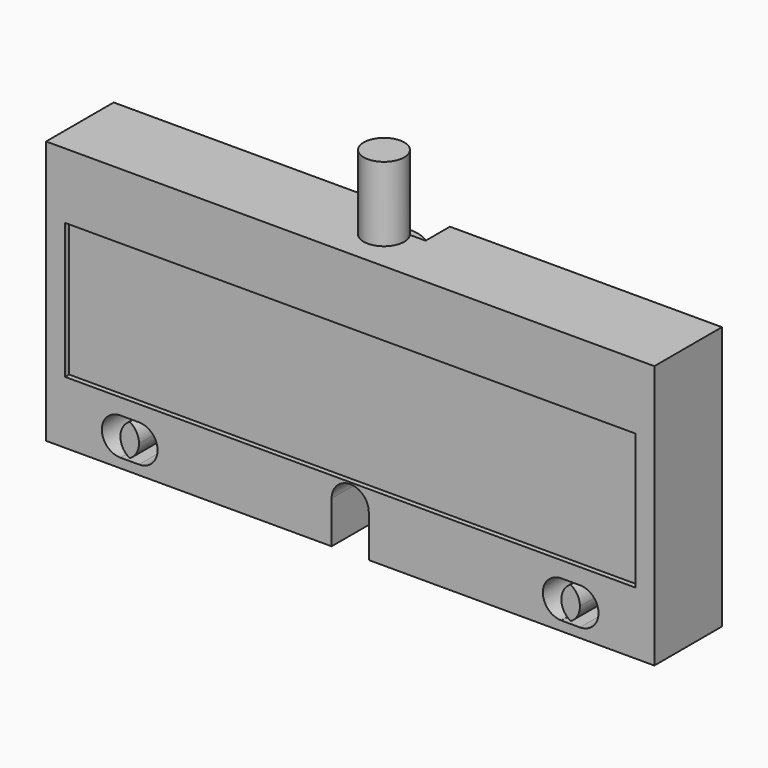
from build123d import *

# Parameters (mm, degrees)
F0_R      = 1.524
F2_DEPTH  = 6.35
F1_R      = 2.54
F3_DEPTH  = 10.16
F4_W      = 45.72
F4_H      = 6.35
F5_DEPTH  = 13.97
F6_DEPTH  = 0.762
F7_DEPTH  = 10.16
F8_DEPTH  = 1.27
F9_DEPTH  = 5.08
F11_DEPTH = 25.4
F12_W     = 21.4504245669
F12_H     = 10.1925823838
F12_W_2   = 21.4354675263
F13_DEPTH = 0.381
F14_W     = 4.826
F14_H     = 20.32
F15_DEPTH = 2.286


with BuildPart() as f2:
    # F0 (on Top) → F2 (new body)
    with BuildSketch(Plane.XY):
        Circle(F0_R)
    extrude(amount=F2_DEPTH)

    # F1 (on Top) → F3 (join)
    with BuildSketch(Plane.XY):
        Circle(F1_R)
    extrude(amount=-F3_DEPTH)


with BuildPart() as f5:
    # F4 (on Top) → F5 (new body)
    with BuildSketch(Plane.XY):
        Rectangle(F4_W, F4_H)
    extrude(amount=-F5_DEPTH)

    # F6 (add): a face of the model
    f6_faces = [f5.faces().sort_by_distance(p)[0] for p in [
        (0, 0, 0),
    ]]
    extrude(f6_faces, amount=F6_DEPTH)

    # F1 (on Top) → F7 (cut)
    with BuildSketch(Plane.XY):
        Circle(F1_R)
    extrude(amount=-F7_DEPTH, mode=Mode.SUBTRACT)

    # F0 (on Top) → F8 (cut)
    with BuildSketch(Plane.XY):
        Circle(F0_R)
    extrude(amount=F8_DEPTH, mode=Mode.SUBTRACT)

    # F9 (add): a face of the model
    f9_faces = [f5.faces().sort_by_distance(p)[0] for p in [
        (0, 0, -13.97),
    ]]
    extrude(f9_faces, amount=F9_DEPTH)

    # F10 (on face) → F11 (cut)
    with BuildSketch(Plane.XZ.offset(3.175)):
        with BuildLine():
            ThreePointArc((-15.875, -18.3439323009), (-14.8871718267, -17.9347604742), (-14.478, -16.9469323009))
            ThreePointArc((-14.478, -16.9469323009), (-14.8871718267, -15.9591041276), (-15.875, -15.5499323009))
            ThreePointArc((-15.875, -15.5499323009), (-16.236570206, -15.5975339216), (-16.5735, -15.7370948118))
            ThreePointArc((-16.5735, -15.7370948118), (-16.0621625109, -16.2484323009), (-15.875, -16.9469323009))
            ThreePointArc((-15.875, -16.9469323009), (-16.0621625109, -17.6454323009), (-16.5735, -18.15676979))
            ThreePointArc((-16.5735, -18.15676979), (-16.236570206, -18.2963306803), (-15.875, -18.3439323009))
        make_face()
        with BuildLine():
            ThreePointArc((-16.5735, -15.7370948118), (-16.236570206, -15.5975339216), (-15.875, -15.5499323009))
            Line((-15.875, -15.5499323009), (-17.272, -15.5499323009))
            ThreePointArc((-17.272, -15.5499323009), (-16.910429794, -15.5975339216), (-16.5735, -15.7370948118))
        make_face()
        with BuildLine():
            Line((-17.272, -18.3439323009), (-15.875, -18.3439323009))
            ThreePointArc((-15.875, -18.3439323009), (-16.236570206, -18.2963306803), (-16.5735, -18.15676979))
            ThreePointArc((-16.5735, -18.15676979), (-16.910429794, -18.2963306803), (-17.272, -18.3439323009))
        make_face()
        with BuildLine():
            ThreePointArc((-16.5735, -18.15676979), (-17.272, -16.9469323009), (-16.5735, -15.7370948118))
            ThreePointArc((-16.5735, -15.7370948118), (-16.910429794, -15.5975339216), (-17.272, -15.5499323009))
            ThreePointArc((-17.272, -15.5499323009), (-18.669, -16.9469323009), (-17.272, -18.3439323009))
            ThreePointArc((-17.272, -18.3439323009), (-16.910429794, -18.2963306803), (-16.5735, -18.15676979))
        make_face()
        with BuildLine():
            Line((17.2682517423, -18.3439323009), (17.2682517423, -16.9469323009))
            ThreePointArc((17.2682517423, -16.9469323009), (17.0805074315, -17.6454323009), (16.5678725715, -18.1556829026))
            ThreePointArc((16.5678725715, -18.1556829026), (16.9056332035, -18.2960493438), (17.2682517423, -18.3439323009))
        make_face()
        with BuildLine():
            ThreePointArc((16.5678725715, -15.7381816992), (17.0805074315, -16.2484323009), (17.2682517423, -16.9469323009))
            Line((17.2682517423, -16.9469323009), (17.2682517423, -15.5536805586))
            Line((17.2682517423, -15.5536805586), (17.1659845309, -15.5536805586))
            ThreePointArc((17.1659845309, -15.5536805586), (16.8564623891, -15.6120021422), (16.5678725715, -15.7381816992))
        make_face()
        with BuildLine():
            Line((17.2682517423, -15.5536805586), (17.2682517423, -16.9469323009))
            Line((17.2682517423, -16.9469323009), (17.2682517423, -18.3439323009))
            ThreePointArc((17.2682517423, -18.3439323009), (18.2560799156, -17.9347604742), (18.6652517423, -16.9469323009))
            ThreePointArc((18.6652517423, -16.9469323009), (18.2192358919, -15.9235857579), (17.1659845309, -15.5536805586))
            Line((17.1659845309, -15.5536805586), (17.2682517423, -15.5536805586))
        make_face()
        with BuildLine():
            ThreePointArc((15.875, -16.8446650895), (16.0842335949, -16.205507978), (16.5678725715, -15.7381816992))
            ThreePointArc((16.5678725715, -15.7381816992), (16.2335083929, -15.6005957347), (15.875, -15.5536805586))
            Line((15.875, -15.5536805586), (15.875, -16.8446650895))
        make_face()
        with BuildLine():
            ThreePointArc((15.875, -15.5536805586), (16.2335083929, -15.6005957347), (16.5678725715, -15.7381816992))
            ThreePointArc((16.5678725715, -15.7381816992), (16.8564623891, -15.6120021422), (17.1659845309, -15.5536805586))
            Line((17.1659845309, -15.5536805586), (15.875, -15.5536805586))
        make_face()
        with BuildLine():
            ThreePointArc((17.2682517423, -18.3439323009), (16.9056332035, -18.2960493438), (16.5678725715, -18.1556829026))
            ThreePointArc((16.5678725715, -18.1556829026), (16.2335083929, -18.2932688672), (15.875, -18.3401840432))
            Line((15.875, -18.3401840432), (15.875, -18.3439323009))
            Line((15.875, -18.3439323009), (17.2682517423, -18.3439323009))
        make_face()
        with BuildLine():
            ThreePointArc((15.875, -18.3401840432), (16.2335083929, -18.2932688672), (16.5678725715, -18.1556829026))
            ThreePointArc((16.5678725715, -18.1556829026), (16.0842335949, -17.6883566239), (15.875, -17.0491995123))
            Line((15.875, -17.0491995123), (15.875, -18.3401840432))
        make_face()
        with BuildLine():
            Line((15.875, -16.8446650895), (15.875, -15.5536805586))
            ThreePointArc((15.875, -15.5536805586), (14.4817482577, -16.9469323009), (15.875, -18.3401840432))
            Line((15.875, -18.3401840432), (15.875, -17.0491995123))
            ThreePointArc((15.875, -17.0491995123), (15.8712517423, -16.9469323009), (15.875, -16.8446650895))
        make_face()
        with BuildLine():
            Line((-1.397, -15.8801323009), (1.397, -15.8801323009))
            ThreePointArc((1.397, -15.8801323009), (0, -14.4831323009), (-1.397, -15.8801323009))
        make_face()
        with BuildLine():
            Line((1.3987992425, -15.8801323009), (1.397, -15.8801323009))
            ThreePointArc((1.397, -15.8801323009), (0, -17.2771323009), (-1.397, -15.8801323009))
            Line((-1.397, -15.8801323009), (-1.397, -20.1916601509))
            Line((-1.397, -20.1916601509), (1.3987992425, -20.1916601509))
            Line((1.3987992425, -20.1916601509), (1.3987992425, -15.8801323009))
        make_face()
        with BuildLine():
            ThreePointArc((-1.397, -15.8801323009), (0, -17.2771323009), (1.397, -15.8801323009))
            Line((1.397, -15.8801323009), (-1.397, -15.8801323009))
        make_face()
    extrude(amount=-F11_DEPTH, mode=Mode.SUBTRACT)

    # F12 (on face) → F13 (cut)
    with BuildSketch(Plane.XZ.offset(3.175)):
        with Locations((10.7252122834, -9.2556457967)):
            Rectangle(F12_W, F12_H)
        with Locations((-10.7177337632, -9.2556457967)):
            Rectangle(F12_W_2, F12_H)
    extrude(amount=-F13_DEPTH, mode=Mode.SUBTRACT)

    # F14 (on face) → F15 (cut)
    with BuildSketch(Plane(origin=(0, 3.175, 0), x_dir=(-1, 0, 0), z_dir=(0, 1, 0))):
        Rectangle(F14_W, F14_H)
    extrude(amount=-F15_DEPTH, mode=Mode.SUBTRACT)


solid = Compound([f2.part, f5.part])
